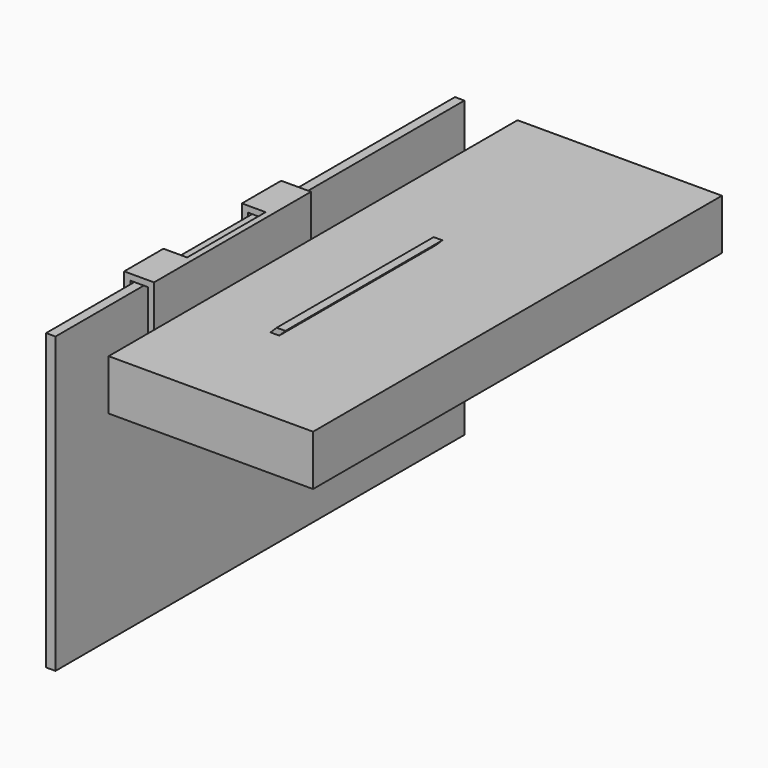
from build123d import *

# Parameters (mm, degrees)
F1_W          = 2.3
F1_H          = 72
F2_DEPTH      = 75
F2_DEPTH_BACK = 50
F3_W          = 50
F3_H          = 12.35
F4_DEPTH      = 75
F4_DEPTH_BACK = 50
F6_DEPTH      = 48
F7_W          = 24
F7_H          = 7.5
F8_DEPTH      = 5.8


with BuildPart() as f2:
    # F1 (on Front) → F2 (new body, two sides)
    with BuildSketch(Plane.XZ) as f2_sk:
        with Locations((-1.15, -36)):
            Rectangle(F1_W, F1_H)
    extrude(amount=F2_DEPTH)
    extrude(f2_sk.sketch, amount=-F2_DEPTH_BACK)


with BuildPart() as f4:
    # F3 (on Front) → F4 (new body, two sides)
    with BuildSketch(Plane.XZ) as f4_sk:
        with Locations((38, -6.175)):
            Rectangle(F3_W, F3_H)
    extrude(amount=F4_DEPTH)
    extrude(f4_sk.sketch, amount=-F4_DEPTH_BACK)


with BuildPart() as f6:
    # F5 (on Front) → F6 (new body)
    with BuildSketch(Plane.XZ):
        Polygon((-4.8, 1.5), (-4.8, -6), (-3.3, -6), (-3.3, 0), (1, 0), (1, -26.1228512973), (3.9992345232, -29.1220858204), (34.6213203436, 1.5), (32.5, 1.5), (3.9992345232, -27.0007654768), (2.5, -25.5015309537), (2.5, 1.5), align=None)
    extrude(amount=F6_DEPTH)

    # F7 (on face) → F8 (cut, through all)
    with BuildSketch(Plane(origin=(-4.8, 0, 0), x_dir=(0, -1, 0), z_dir=(-1, 0, 0))):
        with Locations((24, -2.25)):
            Rectangle(F7_W, F7_H)
    extrude(amount=-F8_DEPTH, mode=Mode.SUBTRACT)


solid = Compound([f2.part, f4.part, f6.part])
